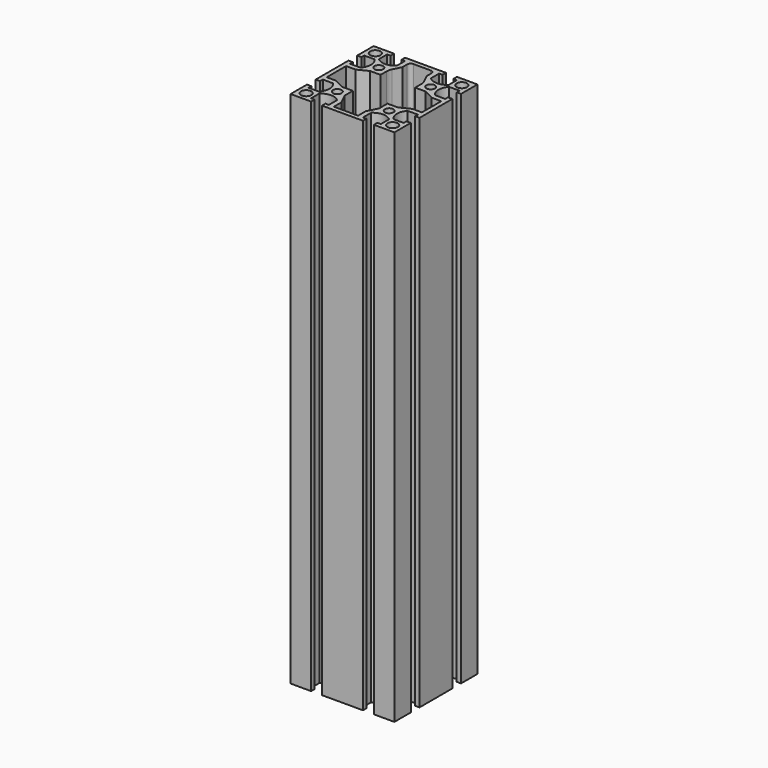
from build123d import *

# Parameters (mm, degrees)
F0_R     = 3
F0_R_2   = 2.5
F1_DEPTH = 300
F2_R     = 2
F3_R     = 7


# Not quite as in the source:
# - a feature names something its author has since deleted; it is built from what else it names


with BuildPart() as f1:
    # F0 (on Top) → F1 (new body)
    with BuildSketch(Plane.XY):
        with BuildLine():
            Line((18.15, -30), (30, -30))
            Line((30, -30), (30, -18.15))
            Line((30, -18.15), (27.5, -18.15))
            Line((27.5, -18.15), (27.5, -20.15))
            Line((27.5, -20.15), (21.5477069044, -20.15))
            ThreePointArc((21.5477069044, -20.15), (19.5, -15), (21.5477069044, -9.85))
            Line((21.5477069044, -9.85), (27.5, -9.85))
            Line((27.5, -9.85), (27.5, -11.85))
            Line((27.5, -11.85), (30, -11.85))
            Line((30, -11.85), (30, 11.85))
            Line((30, 11.85), (27.5, 11.85))
            Line((27.5, 11.85), (27.5, 9.85))
            Line((27.5, 9.85), (21.5477069044, 9.85))
            ThreePointArc((21.5477069044, 9.85), (19.5, 15), (21.5477069044, 20.15))
            Line((21.5477069044, 20.15), (27.5, 20.15))
            Line((27.5, 20.15), (27.5, 18.15))
            Line((27.5, 18.15), (30, 18.15))
            Line((30, 18.15), (30, 30))
            Line((30, 30), (18.15, 30))
            Line((18.15, 30), (18.15, 27.5))
            Line((18.15, 27.5), (20.15, 27.5))
            Line((20.15, 27.5), (20.15, 21.5477069044))
            ThreePointArc((20.15, 21.5477069044), (15, 19.5), (9.85, 21.5477069044))
            Line((9.85, 21.5477069044), (9.85, 27.5))
            Line((9.85, 27.5), (11.85, 27.5))
            Line((11.85, 27.5), (11.85, 30))
            Line((11.85, 30), (-11.85, 30))
            Line((-11.85, 30), (-11.85, 27.5))
            Line((-11.85, 27.5), (-9.85, 27.5))
            Line((-9.85, 27.5), (-9.85, 21.5477069044))
            ThreePointArc((-9.85, 21.5477069044), (-15, 19.5), (-20.15, 21.5477069044))
            Line((-20.15, 21.5477069044), (-20.15, 27.5))
            Line((-20.15, 27.5), (-18.15, 27.5))
            Line((-18.15, 27.5), (-18.15, 30))
            Line((-18.15, 30), (-30, 30))
            Line((-30, 30), (-30, 18.15))
            Line((-30, 18.15), (-27.5, 18.15))
            Line((-27.5, 18.15), (-27.5, 20.15))
            Line((-27.5, 20.15), (-21.5477069044, 20.15))
            ThreePointArc((-21.5477069044, 20.15), (-19.5, 15), (-21.5477069044, 9.85))
            Line((-21.5477069044, 9.85), (-27.5, 9.85))
            Line((-27.5, 9.85), (-27.5, 11.85))
            Line((-27.5, 11.85), (-30, 11.85))
            Line((-30, 11.85), (-30, -11.85))
            Line((-30, -11.85), (-27.5, -11.85))
            Line((-27.5, -11.85), (-27.5, -9.85))
            Line((-27.5, -9.85), (-21.5477069044, -9.85))
            ThreePointArc((-21.5477069044, -9.85), (-19.5, -15), (-21.5477069044, -20.15))
            Line((-21.5477069044, -20.15), (-27.5, -20.15))
            Line((-27.5, -20.15), (-27.5, -18.15))
            Line((-27.5, -18.15), (-30, -18.15))
            Line((-30, -18.15), (-30, -30))
            Line((-30, -30), (-18.15, -30))
            Line((-18.15, -30), (-18.15, -27.5))
            Line((-18.15, -27.5), (-20.15, -27.5))
            Line((-20.15, -27.5), (-20.15, -21.5477069044))
            ThreePointArc((-20.15, -21.5477069044), (-15, -19.5), (-9.85, -21.5477069044))
            Line((-9.85, -21.5477069044), (-9.85, -27.5))
            Line((-9.85, -27.5), (-11.85, -27.5))
            Line((-11.85, -27.5), (-11.85, -30))
            Line((-11.85, -30), (11.85, -30))
            Line((11.85, -30), (11.85, -27.5))
            Line((11.85, -27.5), (9.85, -27.5))
            Line((9.85, -27.5), (9.85, -21.5477069044))
            ThreePointArc((9.85, -21.5477069044), (15, -19.5), (20.15, -21.5477069044))
            Line((20.15, -21.5477069044), (20.15, -27.5))
            Line((20.15, -27.5), (18.15, -27.5))
            Line((18.15, -27.5), (18.15, -30))
        make_face()
        with Locations((-25, -25)):
            Circle(F0_R, mode=Mode.SUBTRACT)
        with Locations((-15, -15)):
            Circle(F0_R_2, mode=Mode.SUBTRACT)
        with Locations((25, -25)):
            Circle(F0_R, mode=Mode.SUBTRACT)
        with Locations((15, -15)):
            Circle(F0_R_2, mode=Mode.SUBTRACT)
        with Locations((-25, 25)):
            Circle(F0_R, mode=Mode.SUBTRACT)
        with Locations((-15, 15)):
            Circle(F0_R_2, mode=Mode.SUBTRACT)
        Polygon((-7, 22), (-7, 27.5), (0, 27.5), (7, 27.5), (7, 22), (10, 16), (10, 10), (16, 10), (22, 7), (27.5, 7), (27.5, 0), (27.5, -7), (22, -7), (16, -10), (10, -10), (10, -16), (7, -22), (7, -27.5), (0, -27.5), (-7, -27.5), (-7, -22), (-10, -16), (-10, -10), (-16, -10), (-22, -7), (-27.5, -7), (-27.5, 0), (-27.5, 7), (-22, 7), (-16, 10), (-10, 10), (-10, 16), align=None, mode=Mode.SUBTRACT)
        with Locations((15, 15)):
            Circle(F0_R_2, mode=Mode.SUBTRACT)
        with Locations((25, 25)):
            Circle(F0_R, mode=Mode.SUBTRACT)
    extrude(amount=F1_DEPTH)

    # F2
    f2_edges = [f1.edges().sort_by_distance(p)[0] for p in [
        (-7, 27.5, 150),
        (7, 27.5, 150),
    ]]
    fillet(f2_edges, radius=F2_R)

    # F3
    f3_edges = [f1.edges().sort_by_distance(p)[0] for p in [
        (-10, 16, 150),
        (10, 16, 150),
    ]]
    fillet(f3_edges, radius=F3_R)


solid = f1.part
